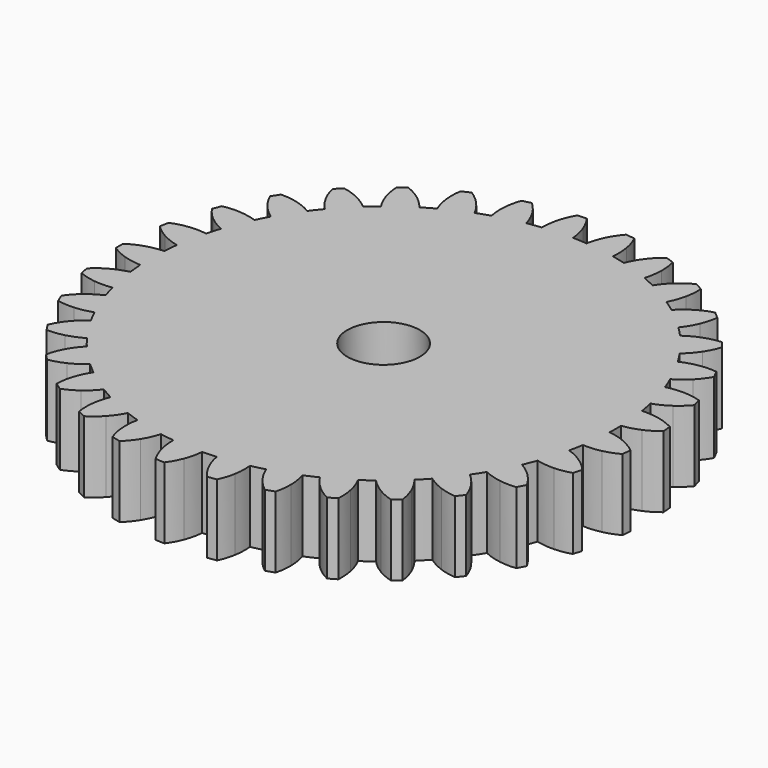
from build123d import *

# Parameters (mm, degrees)
F1_DEPTH  = 5
F2_COUNT  = 33
F3_R      = 2.54
F4_DEPTH  = 1
F5_R      = 1.5
F6_DEPTH  = 1
F7_R      = 2.54
F8_DEPTH  = 4
F9_R      = 1.5
F10_DEPTH = 8


with BuildPart() as f1:
    # F0 (on Top) → F1 (new body)
    with BuildSketch(Plane.XY):
        with BuildLine():
            ThreePointArc((-1.8233572605, 16.1354794051), (-10.8182792774, -12.1096309113), (16.238175, 0))
            ThreePointArc((16.238175, 0), (11.5811549349, 11.3822307877), (0.2813106722, 16.2357380995))
            ThreePointArc((0.2813106722, 16.2357380995), (-0.7726511966, 16.2197822877), (-1.8233572605, 16.1354794051))
        make_face()
        with BuildLine():
            ThreePointArc((-1.8233572605, 16.1354794051), (-0.7726511966, 16.2197822877), (0.2813106722, 16.2357380995))
            ThreePointArc((0.2813106722, 16.2357380995), (0.18304777, 16.8588401245), (0, 17.4625))
            ThreePointArc((0, 17.4625), (-0.2474169209, 17.9997398777), (-0.5655469096, 18.4983731389))
            ThreePointArc((-0.5655469096, 18.4983731389), (-0.880518131, 18.4841652322), (-1.1954136706, 18.4683685865))
            ThreePointArc((-1.1954136706, 18.4683685865), (-1.4647045359, 17.941752741), (-1.6599327052, 17.3834268677))
            ThreePointArc((-1.6599327052, 17.3834268677), (-1.7847695128, 16.7651004952), (-1.8233572605, 16.1354794051))
        make_face()
    extrude(amount=F1_DEPTH)


with BuildPart() as f2_1:
    # F2: instance of F1
    add(f1.part.rotate(Axis((0, 0, 0), (0, 0, -1)), 1 * 360 / F2_COUNT))


with BuildPart() as f2_2:
    # F2: instance of F1
    add(f1.part.rotate(Axis((0, 0, 0), (0, 0, -1)), 2 * 360 / F2_COUNT))


with BuildPart() as f2_3:
    # F2: instance of F1
    add(f1.part.rotate(Axis((0, 0, 0), (0, 0, -1)), 3 * 360 / F2_COUNT))


with BuildPart() as f2_4:
    # F2: instance of F1
    add(f1.part.rotate(Axis((0, 0, 0), (0, 0, -1)), 4 * 360 / F2_COUNT))


with BuildPart() as f2_5:
    # F2: instance of F1
    add(f1.part.rotate(Axis((0, 0, 0), (0, 0, -1)), 5 * 360 / F2_COUNT))


with BuildPart() as f2_6:
    # F2: instance of F1
    add(f1.part.rotate(Axis((0, 0, 0), (0, 0, -1)), 6 * 360 / F2_COUNT))


with BuildPart() as f2_7:
    # F2: instance of F1
    add(f1.part.rotate(Axis((0, 0, 0), (0, 0, -1)), 7 * 360 / F2_COUNT))


with BuildPart() as f2_8:
    # F2: instance of F1
    add(f1.part.rotate(Axis((0, 0, 0), (0, 0, -1)), 8 * 360 / F2_COUNT))


with BuildPart() as f2_9:
    # F2: instance of F1
    add(f1.part.rotate(Axis((0, 0, 0), (0, 0, -1)), 9 * 360 / F2_COUNT))


with BuildPart() as f2_10:
    # F2: instance of F1
    add(f1.part.rotate(Axis((0, 0, 0), (0, 0, -1)), 10 * 360 / F2_COUNT))


with BuildPart() as f2_11:
    # F2: instance of F1
    add(f1.part.rotate(Axis((0, 0, 0), (0, 0, -1)), 11 * 360 / F2_COUNT))


with BuildPart() as f2_12:
    # F2: instance of F1
    add(f1.part.rotate(Axis((0, 0, 0), (0, 0, -1)), 12 * 360 / F2_COUNT))


with BuildPart() as f2_13:
    # F2: instance of F1
    add(f1.part.rotate(Axis((0, 0, 0), (0, 0, -1)), 13 * 360 / F2_COUNT))


with BuildPart() as f2_14:
    # F2: instance of F1
    add(f1.part.rotate(Axis((0, 0, 0), (0, 0, -1)), 14 * 360 / F2_COUNT))


with BuildPart() as f2_15:
    # F2: instance of F1
    add(f1.part.rotate(Axis((0, 0, 0), (0, 0, -1)), 15 * 360 / F2_COUNT))


with BuildPart() as f2_16:
    # F2: instance of F1
    add(f1.part.rotate(Axis((0, 0, 0), (0, 0, -1)), 16 * 360 / F2_COUNT))


with BuildPart() as f2_17:
    # F2: instance of F1
    add(f1.part.rotate(Axis((0, 0, 0), (0, 0, -1)), 17 * 360 / F2_COUNT))


with BuildPart() as f2_18:
    # F2: instance of F1
    add(f1.part.rotate(Axis((0, 0, 0), (0, 0, -1)), 18 * 360 / F2_COUNT))


with BuildPart() as f2_19:
    # F2: instance of F1
    add(f1.part.rotate(Axis((0, 0, 0), (0, 0, -1)), 19 * 360 / F2_COUNT))


with BuildPart() as f2_20:
    # F2: instance of F1
    add(f1.part.rotate(Axis((0, 0, 0), (0, 0, -1)), 20 * 360 / F2_COUNT))


with BuildPart() as f2_21:
    # F2: instance of F1
    add(f1.part.rotate(Axis((0, 0, 0), (0, 0, -1)), 21 * 360 / F2_COUNT))


with BuildPart() as f2_22:
    # F2: instance of F1
    add(f1.part.rotate(Axis((0, 0, 0), (0, 0, -1)), 22 * 360 / F2_COUNT))


with BuildPart() as f2_23:
    # F2: instance of F1
    add(f1.part.rotate(Axis((0, 0, 0), (0, 0, -1)), 23 * 360 / F2_COUNT))


with BuildPart() as f2_24:
    # F2: instance of F1
    add(f1.part.rotate(Axis((0, 0, 0), (0, 0, -1)), 24 * 360 / F2_COUNT))


with BuildPart() as f2_25:
    # F2: instance of F1
    add(f1.part.rotate(Axis((0, 0, 0), (0, 0, -1)), 25 * 360 / F2_COUNT))


with BuildPart() as f2_26:
    # F2: instance of F1
    add(f1.part.rotate(Axis((0, 0, 0), (0, 0, -1)), 26 * 360 / F2_COUNT))


with BuildPart() as f2_27:
    # F2: instance of F1
    add(f1.part.rotate(Axis((0, 0, 0), (0, 0, -1)), 27 * 360 / F2_COUNT))


with BuildPart() as f2_28:
    # F2: instance of F1
    add(f1.part.rotate(Axis((0, 0, 0), (0, 0, -1)), 28 * 360 / F2_COUNT))


with BuildPart() as f2_29:
    # F2: instance of F1
    add(f1.part.rotate(Axis((0, 0, 0), (0, 0, -1)), 29 * 360 / F2_COUNT))


with BuildPart() as f2_30:
    # F2: instance of F1
    add(f1.part.rotate(Axis((0, 0, 0), (0, 0, -1)), 30 * 360 / F2_COUNT))


with BuildPart() as f2_31:
    # F2: instance of F1
    add(f1.part.rotate(Axis((0, 0, 0), (0, 0, -1)), 31 * 360 / F2_COUNT))


with BuildPart() as f2_32:
    # F2: instance of F1
    add(f1.part.rotate(Axis((0, 0, 0), (0, 0, -1)), 32 * 360 / F2_COUNT))


with BuildPart() as f1_1:
    add(f1.part)

    add(f2_1.part)  # F4 merges F2_1

    add(f2_2.part)  # F4 merges F2_2

    add(f2_3.part)  # F4 merges F2_3

    add(f2_4.part)  # F4 merges F2_4

    add(f2_5.part)  # F4 merges F2_5

    add(f2_6.part)  # F4 merges F2_6

    add(f2_7.part)  # F4 merges F2_7

    add(f2_8.part)  # F4 merges F2_8

    add(f2_9.part)  # F4 merges F2_9

    add(f2_10.part)  # F4 merges F2_10

    add(f2_11.part)  # F4 merges F2_11

    add(f2_12.part)  # F4 merges F2_12

    add(f2_13.part)  # F4 merges F2_13

    add(f2_14.part)  # F4 merges F2_14

    add(f2_15.part)  # F4 merges F2_15

    add(f2_16.part)  # F4 merges F2_16

    add(f2_17.part)  # F4 merges F2_17

    add(f2_18.part)  # F4 merges F2_18

    add(f2_19.part)  # F4 merges F2_19

    add(f2_20.part)  # F4 merges F2_20

    add(f2_21.part)  # F4 merges F2_21

    add(f2_22.part)  # F4 merges F2_22

    add(f2_23.part)  # F4 merges F2_23

    add(f2_24.part)  # F4 merges F2_24

    add(f2_25.part)  # F4 merges F2_25

    add(f2_26.part)  # F4 merges F2_26

    add(f2_27.part)  # F4 merges F2_27

    add(f2_28.part)  # F4 merges F2_28

    add(f2_29.part)  # F4 merges F2_29

    add(f2_30.part)  # F4 merges F2_30

    add(f2_31.part)  # F4 merges F2_31

    add(f2_32.part)  # F4 merges F2_32
    # F3 (on face) → F4 (join)
    with BuildSketch(Plane.XY.offset(5)):
        Circle(F3_R)
    extrude(amount=F4_DEPTH)

    # F5 (on face) → F6 (join)
    with BuildSketch(Plane(origin=(0, 0, 0), x_dir=(1, 0, 0), z_dir=(0, 0, -1))):
        Circle(F5_R)
    extrude(amount=F6_DEPTH)

    # F7 (on face) → F8 (cut)
    with BuildSketch(Plane.XY.offset(6)):
        Circle(F7_R)
    extrude(amount=-F8_DEPTH, mode=Mode.SUBTRACT)

    # F9 (on face) → F10 (cut)
    with BuildSketch(Plane(origin=(0, 0, -1), x_dir=(1, 0, 0), z_dir=(0, 0, -1))):
        Circle(F9_R)
    extrude(amount=-F10_DEPTH, mode=Mode.SUBTRACT)


solid = f1_1.part
